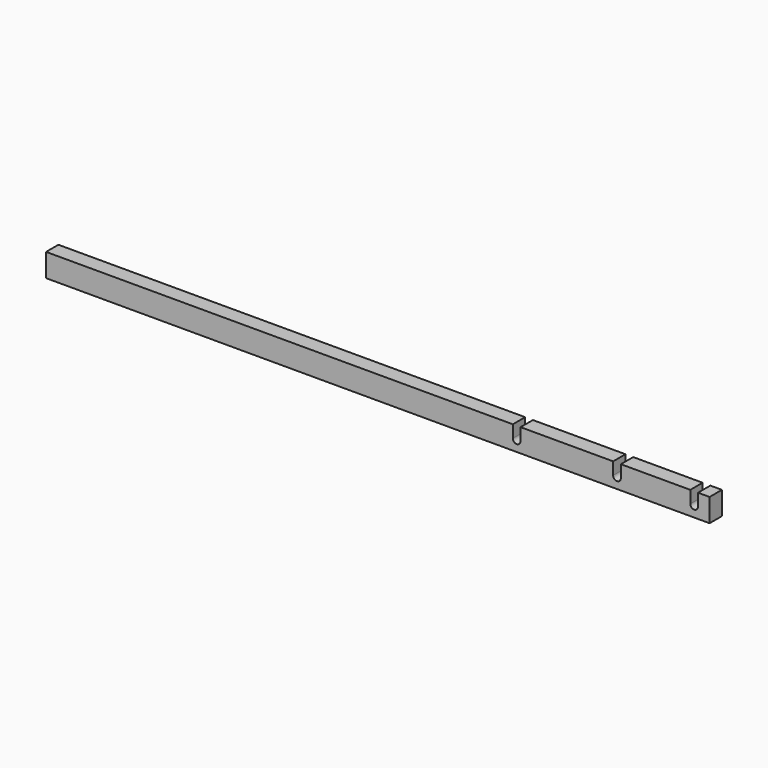
from build123d import *

# Parameters (mm, degrees)
F0_W     = 546.1
F0_H     = 19.05
F1_DEPTH = 12.7
F3_DEPTH = 25.4


# Not quite as in the source:
# - a feature names something its author has since deleted; it is built from what else it names


with BuildPart() as f1:
    # F0 (on Front) → F1 (new body)
    with BuildSketch(Plane.XZ):
        with Locations((196.914867598, 2.5221339893)):
            Rectangle(F0_W, F0_H)
    extrude(amount=F1_DEPTH)

    # F2 (on face) → F3 (cut)
    with BuildSketch(Plane.XZ.offset(12.7)):
        with BuildLine():
            ThreePointArc((390.589867598, 1.8871339893), (393.764867598, 5.0621339893), (396.939867598, 1.8871339893))
            Line((396.939867598, 1.8871339893), (396.939867598, 12.0471339893))
            Line((396.939867598, 12.0471339893), (390.589867598, 12.0471339893))
            Line((390.589867598, 12.0471339893), (390.589867598, 1.8871339893))
        make_face()
        with BuildLine():
            ThreePointArc((390.589867598, 1.8871339893), (393.764867598, -1.2878660107), (396.939867598, 1.8871339893))
            ThreePointArc((396.939867598, 1.8871339893), (393.764867598, 5.0621339893), (390.589867598, 1.8871339893))
        make_face()
        with BuildLine():
            Line((460.439867598, 12.0471339893), (454.089867598, 12.0471339893))
            Line((454.089867598, 12.0471339893), (454.089867598, 1.8871339893))
            ThreePointArc((454.089867598, 1.8871339893), (457.264867598, 5.0621339893), (460.439867598, 1.8871339893))
            Line((460.439867598, 1.8871339893), (460.439867598, 12.0471339893))
        make_face()
        with BuildLine():
            ThreePointArc((460.439867598, 1.8871339893), (457.264867598, 5.0621339893), (454.089867598, 1.8871339893))
            ThreePointArc((454.089867598, 1.8871339893), (457.264867598, -1.2878660107), (460.439867598, 1.8871339893))
        make_face()
        with BuildLine():
            ThreePointArc((308.039867598, 1.8871339893), (311.214867598, -1.2878660107), (314.389867598, 1.8871339893))
            ThreePointArc((314.389867598, 1.8871339893), (311.214867598, 5.0621339893), (308.039867598, 1.8871339893))
        make_face()
        with BuildLine():
            Line((314.389867598, 1.8871339893), (314.389867598, 12.0471339893))
            Line((314.389867598, 12.0471339893), (308.039867598, 12.0471339893))
            Line((308.039867598, 12.0471339893), (308.039867598, 1.8871339893))
            ThreePointArc((308.039867598, 1.8871339893), (311.214867598, 5.0621339893), (314.389867598, 1.8871339893))
        make_face()
    extrude(amount=-F3_DEPTH, mode=Mode.SUBTRACT)


solid = f1.part
